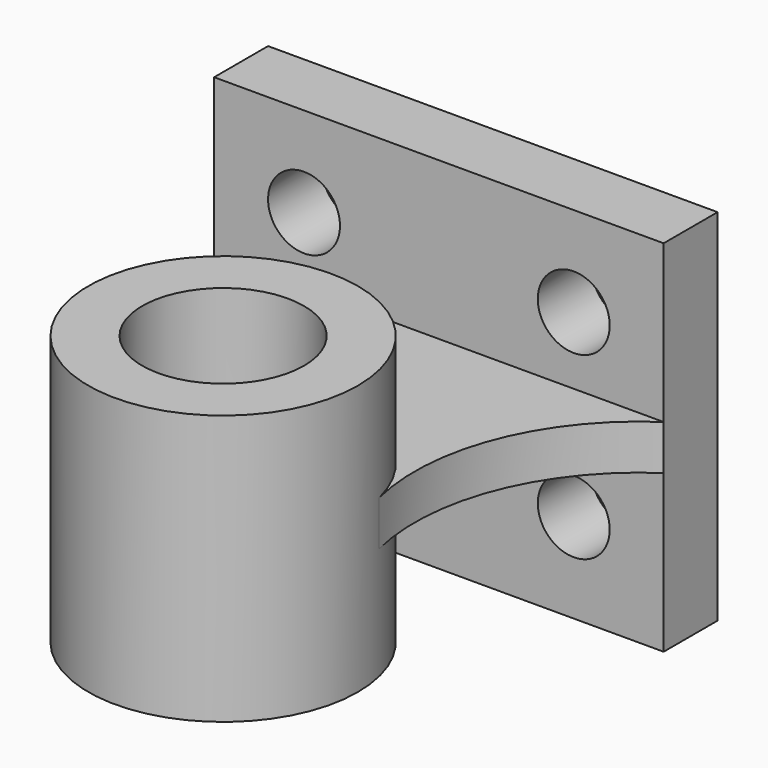
from build123d import *

# Parameters (mm, degrees)
F0_W     = 100
F0_H     = 80
F0_R     = 8
F1_DEPTH = 15
F3_R     = 30
F3_R_2   = 18
F4_DEPTH = 30
F6_DEPTH = 5


# Not quite as in the source:
# - a feature of the source that left no trace in its solid (it failed there, or was rolled back) is left out


with BuildPart() as f1:
    # F0 (on Front) → F1 (new body)
    with BuildSketch(Plane.XZ):
        Rectangle(F0_W, F0_H)
        with Locations((-30, -20)):
            Circle(F0_R, mode=Mode.SUBTRACT)
        with Locations((30, -20)):
            Circle(F0_R, mode=Mode.SUBTRACT)
        with Locations((-30, 20)):
            Circle(F0_R, mode=Mode.SUBTRACT)
        with Locations((30, 20)):
            Circle(F0_R, mode=Mode.SUBTRACT)
    extrude(amount=F1_DEPTH)


with BuildPart() as f4:
    # F3 (on offset) → F4 (new body, symmetric)
    with BuildSketch(Plane(origin=(0, 0, 0), x_dir=(1, 0, 0), z_dir=(0, 0, -1))):
        with Locations((0, 75)):
            Circle(F3_R)
        with Locations((0, 75)):
            Circle(F3_R_2, mode=Mode.SUBTRACT)
    extrude(amount=F4_DEPTH, both=True)


with BuildPart() as f6:
    # F5 (on Top) → F6 (new body, symmetric)
    with BuildSketch(Plane.XY):
        with BuildLine():
            ThreePointArc((29.1897496686, -68.0747913905), (31.2896610375, -38.2809801044), (50, -15))
            Line((50, -15), (-50, -15))
            ThreePointArc((-50, -15), (-31.2896610375, -38.2809801044), (-29.1897496686, -68.0747913905))
            ThreePointArc((-29.1897496686, -68.0747913905), (0, -45), (29.1897496686, -68.0747913905))
        make_face()
    extrude(amount=F6_DEPTH, both=True)


solid = Compound([f1.part, f4.part, f6.part])
